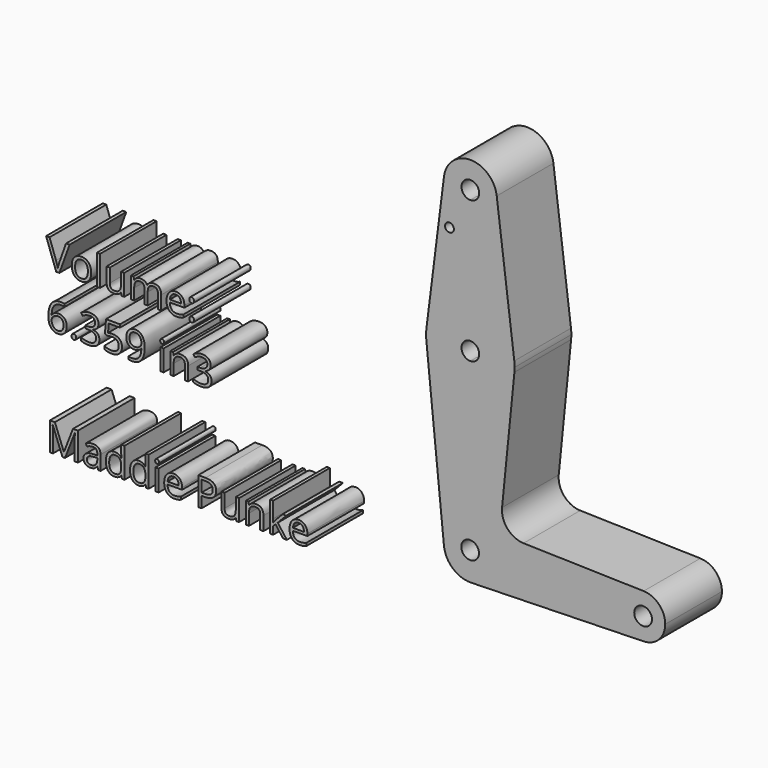
from build123d import *

# Parameters (mm, degrees)
F0_R         = 1.5875
F0_TEXT_SIZE = 14.1449298503
F1_DEPTH     = 25.4


# Not quite as in the source:
# - Text() gives the source's letters only with a copy of the font that has no kerning and outlines rounded to 1/6400 em; it was checked with that copy


with BuildPart() as f1:
    # F0 (on Front) → F1 (new body)
    with BuildSketch(Plane.XZ):
        with BuildLine():
            ThreePointArc((-11.8924484451, 75.2708331202), (-9.5859054809, 67.7800128107), (-2.4421554809, 64.5552081202))
            ThreePointArc((-2.4421554809, 64.5552081202), (4.2930366099, 67.3450160294), (7.0828445191, 74.0802081202))
            ThreePointArc((7.0828445191, 74.0802081202), (7.0641494133, 74.6766913621), (7.0081374833, 75.2708331202))
            ThreePointArc((7.0081374833, 75.2708331202), (-2.4421554809, 83.6052081202), (-11.8924484451, 75.2708331202))
        make_face()
        with BuildLine():
            ThreePointArc((0.7328445191, 74.0802081202), (-0.1970914506, 71.8351440899), (-2.4421554809, 70.9052081202))
            ThreePointArc((-2.4421554809, 70.9052081202), (-4.6872195112, 76.3252721504), (0.7328445191, 74.0802081202))
        make_face(mode=Mode.SUBTRACT)
        with BuildLine():
            ThreePointArc((7.0828445191, 74.0802081202), (4.2930366099, 67.3450160294), (-2.4421554809, 64.5552081202))
            Line((-2.4421554809, 64.5552081202), (-2.4421554809, 39.1552081202))
            ThreePointArc((-2.4421554809, 39.1552081202), (8.0581700349, 35.1864581202), (13.3083327928, 25.2645831202))
            Line((13.3083327928, 25.2645831202), (7.0081374833, 75.2708331202))
            ThreePointArc((7.0081374833, 75.2708331202), (7.0641494133, 74.6766913621), (7.0828445191, 74.0802081202))
        make_face()
        with BuildLine():
            Line((-2.4421554809, 39.1552081202), (-2.4421554809, 64.5552081202))
            ThreePointArc((-2.4421554809, 64.5552081202), (-9.5859054809, 67.7800128107), (-11.8924484451, 75.2708331202))
            Line((-11.8924484451, 75.2708331202), (-18.1926437546, 25.2645831202))
            ThreePointArc((-18.1926437546, 25.2645831202), (-12.9424809967, 35.1864581202), (-2.4421554809, 39.1552081202))
        make_face()
        with Locations((-9.925160557, 59.8054081202)):
            Circle(F0_R, mode=Mode.SUBTRACT)
        with BuildLine():
            ThreePointArc((13.3083327928, 25.2645831202), (8.0581700349, 35.1864581202), (-2.4421554809, 39.1552081202))
            Line((-2.4421554809, 39.1552081202), (-2.4421554809, 26.4552081202))
            ThreePointArc((-2.4421554809, 26.4552081202), (-0.1970914506, 25.5252721504), (0.7328445191, 23.2802081202))
            ThreePointArc((0.7328445191, 23.2802081202), (-0.1970914506, 21.0351440899), (-2.4421554809, 20.1052081202))
            Line((-2.4421554809, 20.1052081202), (-2.4421554809, 7.4052081202))
            ThreePointArc((-2.4421554809, 7.4052081202), (8.2071182619, 11.5069930219), (13.3532700832, 21.6927081202))
            ThreePointArc((13.3532700832, 21.6927081202), (13.4129384297, 22.4854615661), (13.4328445191, 23.2802081202))
            ThreePointArc((13.4328445191, 23.2802081202), (13.4016860095, 24.2743468568), (13.3083327928, 25.2645831202))
        make_face()
        with BuildLine():
            Line((-2.4421554809, 26.4552081202), (-2.4421554809, 39.1552081202))
            ThreePointArc((-2.4421554809, 39.1552081202), (-12.9424809967, 35.1864581202), (-18.1926437546, 25.2645831202))
            ThreePointArc((-18.1926437546, 25.2645831202), (-18.3158992964, 23.4799136069), (-18.237581045, 21.6927081202))
            ThreePointArc((-18.237581045, 21.6927081202), (-13.0914292238, 11.5069930219), (-2.4421554809, 7.4052081202))
            Line((-2.4421554809, 7.4052081202), (-2.4421554809, 20.1052081202))
            ThreePointArc((-2.4421554809, 20.1052081202), (-5.6171554809, 23.2802081202), (-2.4421554809, 26.4552081202))
        make_face()
        with BuildLine():
            ThreePointArc((-2.4421554809, 7.4052081202), (-13.0914292238, 11.5069930219), (-18.237581045, 21.6927081202))
            Line((-18.237581045, 21.6927081202), (-11.9194108194, -41.1722918798))
            ThreePointArc((-11.9194108194, -41.1722918798), (-9.5060845399, -33.8302276341), (-2.4421554809, -30.6947918798))
            Line((-2.4421554809, -30.6947918798), (-2.4421554809, 7.4052081202))
        make_face()
        with BuildLine():
            ThreePointArc((13.3532700832, 21.6927081202), (8.2071182619, 11.5069930219), (-2.4421554809, 7.4052081202))
            Line((-2.4421554809, 7.4052081202), (-2.4421554809, -30.6947918798))
            ThreePointArc((-2.4421554809, -30.6947918798), (4.2930366099, -33.484599789), (7.0828445191, -40.2197918798))
            Line((7.0828445191, -40.2197918798), (51.5328445191, -40.2197918798))
            ThreePointArc((51.5328445191, -40.2197918798), (53.930108898, -34.5356300672), (59.6738701601, -32.284901612))
            Line((59.6738701601, -32.284901612), (16.6244546939, -31.1807074035))
            ThreePointArc((16.6244546939, -31.1807074035), (10.8643850868, -28.4902429255), (8.9179568535, -22.4381013112))
            Line((8.9179568535, -22.4381013112), (13.3532700832, 21.6927081202))
        make_face()
        with BuildLine():
            ThreePointArc((-2.4421554809, -30.6947918798), (-9.5060845399, -33.8302276341), (-11.9194108194, -41.1722918798))
            ThreePointArc((-11.9194108194, -41.1722918798), (-8.7406238686, -47.3650645107), (-2.1979247117, -49.7416602013))
            ThreePointArc((-2.1979247117, -49.7416602013), (4.3788386943, -46.8680746252), (7.0828445191, -40.2197918798))
            Line((7.0828445191, -40.2197918798), (0.5805136643, -40.2197918798))
            ThreePointArc((0.5805136643, -40.2197918798), (-5.0183650251, -41.5277864731), (-2.4421554809, -36.3876077973))
            Line((-2.4421554809, -36.3876077973), (-2.4421554809, -30.6947918798))
        make_face()
        with BuildLine():
            ThreePointArc((7.0828445191, -40.2197918798), (4.3788386943, -46.8680746252), (-2.1979247117, -49.7416602013))
            Line((-2.1979247117, -49.7416602013), (59.6738701601, -48.1546821477))
            ThreePointArc((59.6738701601, -48.1546821477), (53.930108898, -45.9039536925), (51.5328445191, -40.2197918798))
            Line((51.5328445191, -40.2197918798), (7.0828445191, -40.2197918798))
        make_face()
        with BuildLine():
            ThreePointArc((51.5328445191, -40.2197918798), (53.930108898, -45.9039536925), (59.6738701601, -48.1546821477))
            ThreePointArc((59.6738701601, -48.1546821477), (65.1545063318, -45.7600275009), (67.4078445191, -40.2197918798))
            ThreePointArc((67.4078445191, -40.2197918798), (65.1545063318, -34.6795562588), (59.6738701601, -32.284901612))
            ThreePointArc((59.6738701601, -32.284901612), (53.930108898, -34.5356300672), (51.5328445191, -40.2197918798))
        make_face()
        with BuildLine():
            ThreePointArc((62.6453445191, -40.2197918798), (59.4703445191, -43.3947918798), (56.2953445191, -40.2197918798))
            ThreePointArc((56.2953445191, -40.2197918798), (59.4703445191, -37.0447918798), (62.6453445191, -40.2197918798))
        make_face(mode=Mode.SUBTRACT)
        with Locations((-154.5175740574, 0)):
            Text('Volume:', F0_TEXT_SIZE, font='Open Sans', text_align=(TextAlign.LEFT, TextAlign.BOTTOM))
        with Locations((-154.5175740574, -19.2371045964)):
            Text('6.359 in3', F0_TEXT_SIZE, font='Open Sans', text_align=(TextAlign.LEFT, TextAlign.BOTTOM))
        with Locations((-154.5175740574, -57.7113137891)):
            Text('Maddie Punke', F0_TEXT_SIZE, font='Open Sans', text_align=(TextAlign.LEFT, TextAlign.BOTTOM))
        with BuildLine():
            ThreePointArc((7.0828445191, -40.2197918798), (4.2930366099, -33.484599789), (-2.4421554809, -30.6947918798))
            Line((-2.4421554809, -30.6947918798), (-2.4421554809, -36.3876077973))
            ThreePointArc((-2.4421554809, -36.3876077973), (-0.2511573984, -37.3461109824), (0.6495041691, -39.5615138113))
            ThreePointArc((0.6495041691, -39.5615138113), (0.6322094393, -39.8924555378), (0.5805136643, -40.2197918798))
            Line((0.5805136643, -40.2197918798), (7.0828445191, -40.2197918798))
        make_face()
    extrude(amount=F1_DEPTH)


solid = f1.part
